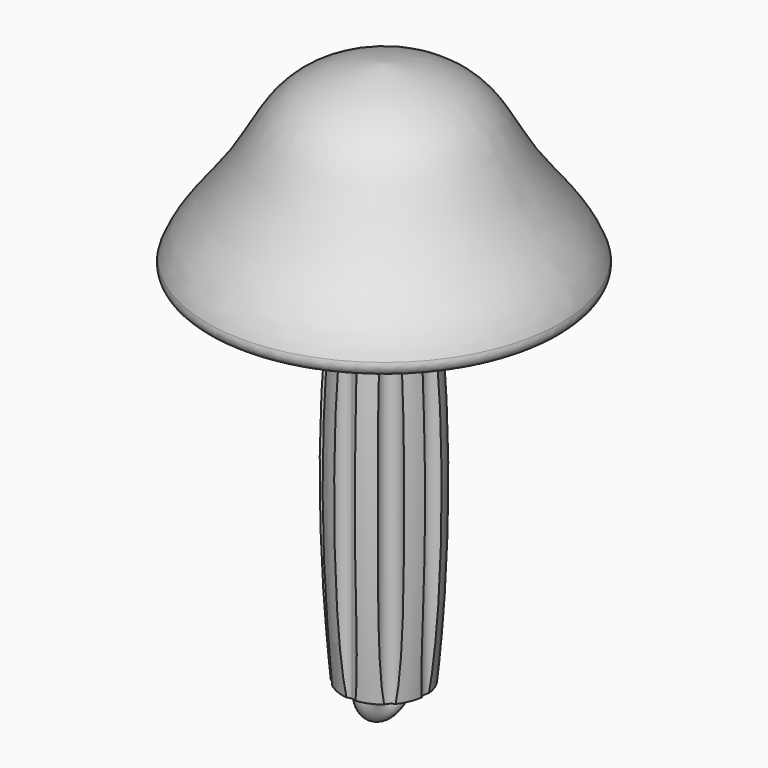
from build123d import *

# Parameters (mm, degrees)
F2_R     = 1.5
F3_R     = 1.375
F4_ANGLE = 180
F5_R     = 1.5
F6_DEPTH = 50
F8_DEPTH = 3


# Not quite as in the source:
# - a feature names something its author has since deleted; it is built from what else it names


with BuildPart() as f1:
    # F0 (on Front) → F1 (revolve)
    with BuildSketch(Plane.XZ):
        with BuildLine():
            Line((0, 69.0493063515), (0, 0))
            Line((0, 0), (6, 0))
            ThreePointArc((6, 0), (7.2926790564, 25.839637965), (6, 51.6792759299))
            Line((6, 51.6792759299), (26, 51.6792759299))
            add(Edge.make_bspline(
                [(26, 51.6792759299), (25.5531692211, 56.0018357257), (17.4177627874, 63.5388246851), (13.1908107993, 75.6280057098), (3.6355278267, 78.1464873003), (0, 78.4764438868)],
                knots=[0, 0, 0, 0, 0.3501423197, 0.6778140823, 1, 1, 1, 1], degree=3))
            Line((0, 78.4764438868), (0, 69.0493063515))
        make_face()
    revolve(axis=Axis((0, 0, 34.5246531758), (0, 0, -1)))

    # F2
    f2_edges = [f1.edges().sort_by_distance(p)[0] for p in [
        (-6, 0, 51.679276),
        (-26, 0, 51.679276),
    ]]
    fillet(f2_edges, radius=F2_R)

    # F3 (on Top) → F4 (revolve)
    with BuildSketch(Plane.XY):
        with Locations((0, -3.5)):
            Circle(F3_R)
    revolve(axis=Axis((7.1852505207, 0, 0), (1, 0, 0)), revolution_arc=F4_ANGLE)

    # F5 (on face) → F6 (cut)
    with BuildSketch(Plane(origin=(0, 0, 0), x_dir=(1, 0, 0), z_dir=(0, 0, -1))):
        with BuildLine():
            ThreePointArc((0, 5.8148366335), (1.0606601718, 6.2541764617), (1.5, 7.3148366335))
            ThreePointArc((1.5, 7.3148366335), (-1.0606601718, 8.3754968053), (0, 5.8148366335))
        make_face()
        with Locations((-5.1723705868, 5.1723705868)):
            Circle(F5_R)
        with Locations((-7.3148366335, 0)):
            Circle(F5_R)
        with Locations((-5.1723705868, -5.1723705868)):
            Circle(F5_R)
        with Locations((0, -7.3148366335)):
            Circle(F5_R)
        with Locations((5.1723705868, -5.1723705868)):
            Circle(F5_R)
        with Locations((7.3148366335, 0)):
            Circle(F5_R)
        with Locations((5.1723705868, 5.1723705868)):
            Circle(F5_R)
    extrude(amount=-F6_DEPTH, mode=Mode.SUBTRACT)

    # F7 (on face) → F8 (cut)
    with BuildSketch(Plane(origin=(0, 0, 51.6792759299), x_dir=(1, 0, 0), z_dir=(0, 0, -1))):
        with BuildLine():
            ThreePointArc((-0.8801164986, 8.3737491301), (0, 8.4198740813), (0.8801164986, 8.3737491301))
            Line((0.8801164986, 8.3737491301), (2.3456272357, 22.3171523937))
            ThreePointArc((2.3456272357, 22.3171523937), (0, 22.4400815082), (-2.3456272357, 22.3171523937))
            Line((-2.3456272357, 22.3171523937), (-0.8801164986, 8.3737491301))
        make_face()
        with BuildLine():
            Line((-3.424671319, 7.6919377209), (-9.127203423, 20.5000345309))
            ThreePointArc((-9.127203423, 20.5000345309), (-11.2200407541, 19.4336806491), (-13.1899489708, 18.1544072953))
            Line((-13.1899489708, 18.1544072953), (-4.9490778112, 6.8118212223))
            ThreePointArc((-4.9490778112, 6.8118212223), (-4.2099370407, 7.2918248511), (-3.424671319, 7.6919377209))
        make_face()
        with BuildLine():
            Line((-6.8118212223, 4.9490778112), (-18.1544072953, 13.1899489708))
            ThreePointArc((-18.1544072953, 13.1899489708), (-19.4336806491, 11.2200407541), (-20.5000345309, 9.127203423))
            Line((-20.5000345309, 9.127203423), (-7.6919377209, 3.424671319))
            ThreePointArc((-7.6919377209, 3.424671319), (-7.2918248511, 4.2099370407), (-6.8118212223, 4.9490778112))
        make_face()
        with BuildLine():
            Line((-8.3737491301, 0.8801164986), (-22.3171523937, 2.3456272357))
            ThreePointArc((-22.3171523937, 2.3456272357), (-22.4400815082, 0), (-22.3171523937, -2.3456272357))
            Line((-22.3171523937, -2.3456272357), (-8.3737491301, -0.8801164986))
            ThreePointArc((-8.3737491301, -0.8801164986), (-8.4198740813, 0), (-8.3737491301, 0.8801164986))
        make_face()
        with BuildLine():
            Line((-7.6919377209, -3.424671319), (-20.5000345309, -9.127203423))
            ThreePointArc((-20.5000345309, -9.127203423), (-19.4336806491, -11.2200407541), (-18.1544072953, -13.1899489708))
            Line((-18.1544072953, -13.1899489708), (-6.8118212223, -4.9490778112))
            ThreePointArc((-6.8118212223, -4.9490778112), (-7.2918248511, -4.2099370407), (-7.6919377209, -3.424671319))
        make_face()
        with BuildLine():
            Line((-4.9490778112, -6.8118212223), (-13.1899489708, -18.1544072953))
            ThreePointArc((-13.1899489708, -18.1544072953), (-11.2200407541, -19.4336806491), (-9.127203423, -20.5000345309))
            Line((-9.127203423, -20.5000345309), (-3.424671319, -7.6919377209))
            ThreePointArc((-3.424671319, -7.6919377209), (-4.2099370407, -7.2918248511), (-4.9490778112, -6.8118212223))
        make_face()
        with BuildLine():
            Line((-0.8801164986, -8.3737491301), (-2.3456272357, -22.3171523937))
            ThreePointArc((-2.3456272357, -22.3171523937), (0, -22.4400815082), (2.3456272357, -22.3171523937))
            Line((2.3456272357, -22.3171523937), (0.8801164986, -8.3737491301))
            ThreePointArc((0.8801164986, -8.3737491301), (0, -8.4198740813), (-0.8801164986, -8.3737491301))
        make_face()
        with BuildLine():
            Line((3.424671319, -7.6919377209), (9.127203423, -20.5000345309))
            ThreePointArc((9.127203423, -20.5000345309), (11.2200407541, -19.4336806491), (13.1899489708, -18.1544072953))
            Line((13.1899489708, -18.1544072953), (4.9490778112, -6.8118212223))
            ThreePointArc((4.9490778112, -6.8118212223), (4.2099370407, -7.2918248511), (3.424671319, -7.6919377209))
        make_face()
        with BuildLine():
            Line((6.8118212223, -4.9490778112), (18.1544072953, -13.1899489708))
            ThreePointArc((18.1544072953, -13.1899489708), (19.4336806491, -11.2200407541), (20.5000345309, -9.127203423))
            Line((20.5000345309, -9.127203423), (7.6919377209, -3.424671319))
            ThreePointArc((7.6919377209, -3.424671319), (7.2918248511, -4.2099370407), (6.8118212223, -4.9490778112))
        make_face()
        with BuildLine():
            Line((8.3737491301, -0.8801164986), (22.3171523937, -2.3456272357))
            ThreePointArc((22.3171523937, -2.3456272357), (22.4400815082, 0), (22.3171523937, 2.3456272357))
            Line((22.3171523937, 2.3456272357), (8.3737491301, 0.8801164986))
            ThreePointArc((8.3737491301, 0.8801164986), (8.4198740813, 0), (8.3737491301, -0.8801164986))
        make_face()
        with BuildLine():
            Line((7.6919377209, 3.424671319), (20.5000345309, 9.127203423))
            ThreePointArc((20.5000345309, 9.127203423), (19.4336806491, 11.2200407541), (18.1544072953, 13.1899489708))
            Line((18.1544072953, 13.1899489708), (6.8118212223, 4.9490778112))
            ThreePointArc((6.8118212223, 4.9490778112), (7.2918248511, 4.2099370407), (7.6919377209, 3.424671319))
        make_face()
        with BuildLine():
            Line((4.9490778112, 6.8118212223), (13.1899489708, 18.1544072953))
            ThreePointArc((13.1899489708, 18.1544072953), (11.2200407541, 19.4336806491), (9.127203423, 20.5000345309))
            Line((9.127203423, 20.5000345309), (3.424671319, 7.6919377209))
            ThreePointArc((3.424671319, 7.6919377209), (4.2099370407, 7.2918248511), (4.9490778112, 6.8118212223))
        make_face()
    extrude(amount=-F8_DEPTH, mode=Mode.SUBTRACT)


solid = f1.part
